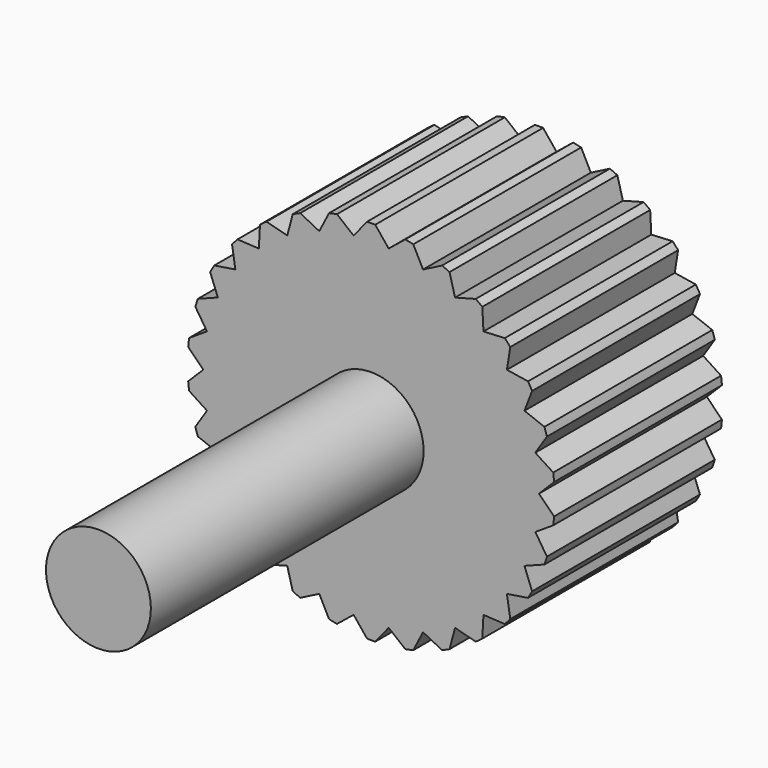
from build123d import *

# Parameters (mm, degrees)
F0_R            = 1
F1_DEPTH        = 6.5
F2_R            = 3.5
F3_DEPTH        = 4
F5_DEPTH        = 10.501
F5_COPIES_COUNT = 30


# Not quite as in the source:
# - a pattern or mirror of a feature is missing from the dataset's text; its kind, count and spacing are read off the source's solid


with BuildPart() as f1:
    # F0 (on Front) → F1 (new body)
    with BuildSketch(Plane.XZ):
        Circle(F0_R)
    extrude(amount=F1_DEPTH)

    # F2 (on face) → F3 (join)
    with BuildSketch(Plane(origin=(0, 0, 0), x_dir=(-1, 0, 0), z_dir=(0, 1, 0))):
        Circle(F2_R)
    extrude(amount=F3_DEPTH)

    # F4 (on face) → F5 (cut, through all)
    with BuildSketch(Plane(origin=(0, 4, 0), x_dir=(-1, 0, 0), z_dir=(0, 1, 0))):
        with BuildLine():
            Line((3.2, 0), (3.4881207588, -0.2881207588))
            ThreePointArc((3.4881207588, -0.2881207588), (3.5, 0), (3.4881207588, 0.2881207588))
            Line((3.4881207588, 0.2881207588), (3.2, 0))
        make_face()
    f5 = extrude(amount=-F5_DEPTH, mode=Mode.SUBTRACT)

    # F5_copies: F5 ×30 about axis
    f5_copies_axis = Axis((0, 0, 0), (0, 1, 0))
    for i in range(1, F5_COPIES_COUNT):
        add(f5.rotate(f5_copies_axis, i * 360 / F5_COPIES_COUNT), mode=Mode.SUBTRACT)


solid = f1.part
